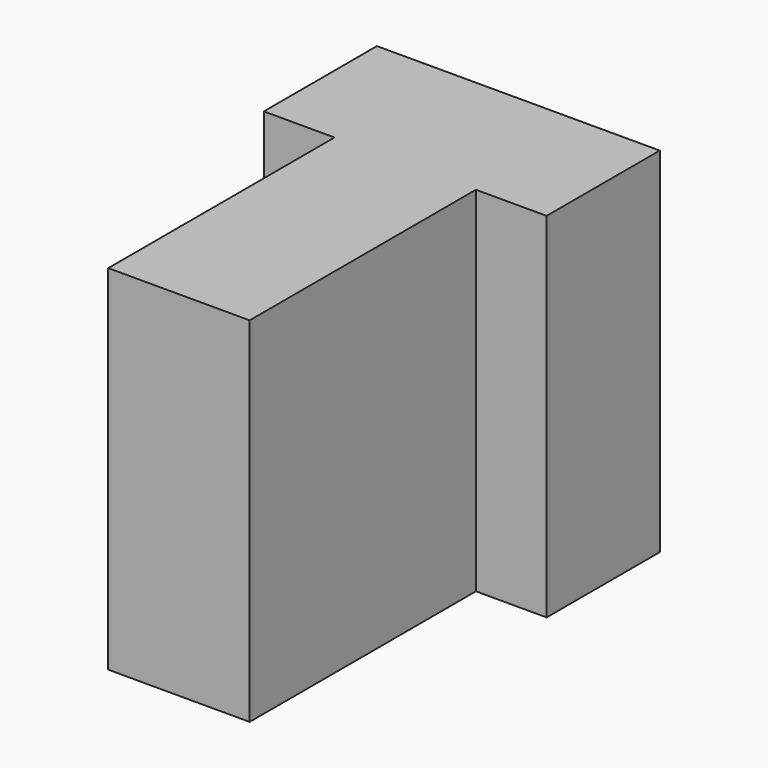
from build123d import *

# Parameters (mm, degrees)
F1_DEPTH = 31.75


# Not quite as in the source:
# - a length typed as a fraction of an inch, garbled in the dataset ("3 / 203.2 mm" for 3/8 in), is restored


with BuildPart() as f1:
    # F0 (on Top) → F1 (new body)
    with BuildSketch(Plane.XY):
        Polygon((13.946997959, 26.0384509316), (-11.453002041, 26.0384509316), (-11.453002041, 13.3384509316), (-5.103002041, 13.3384509316), (-5.103002041, -12.0615490684), (7.596997959, -12.0615490684), (7.596997959, 13.3384509316), (13.946997959, 13.3384509316), align=None)
    extrude(amount=F1_DEPTH)


solid = f1.part
